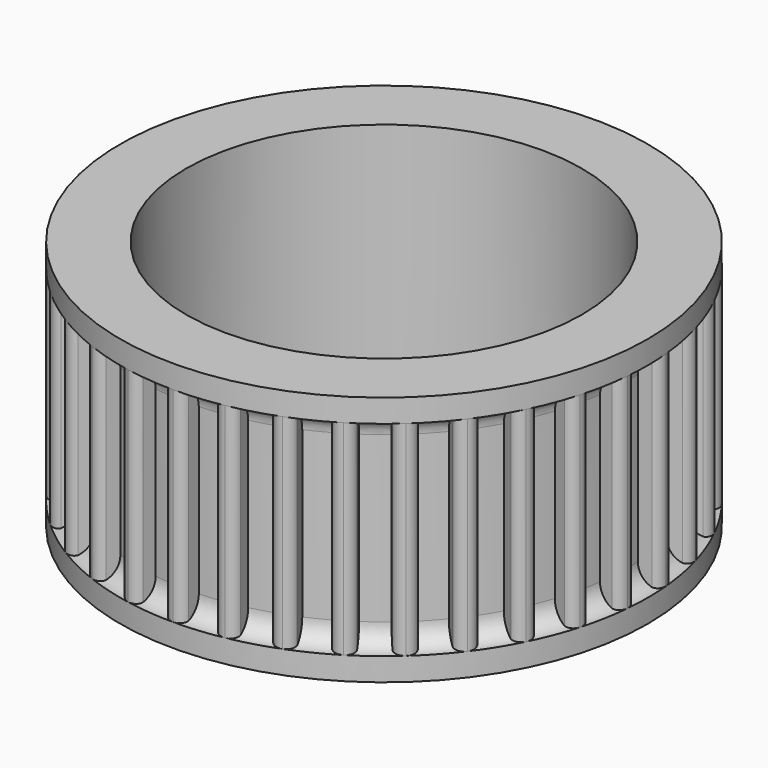
from build123d import *

# Parameters (mm, degrees)
F0_R             = 20
F1_DEPTH         = 19
F2_W             = 1.5
F2_H             = 15.5
F5_R             = 1.49999
F4_W             = 1.5
F4_H             = 19.3690806627
F6_DEPTH         = 19
F6_COPIES_COUNT  = 34
F6_COPIES1_COUNT = 2
F6_COPIES1_ANGLE = 84.7059
F6_COPIES2_COUNT = 2
F6_COPIES2_ANGLE = 95.2941
F6_COPIES3_COUNT = 2
F6_COPIES3_ANGLE = 275.2941
F7_R             = 15
F8_DEPTH         = 19.001


# Not quite as in the source:
# - a fillet or chamfer is up to 0.001 mm smaller than in the source, because OpenCascade refuses the exact size
# - a pattern or mirror of a feature is missing from the dataset's text; its kind, count and spacing are read off the source's solid


with BuildPart() as f1:
    # F0 (on Top) → F1 (new body)
    with BuildSketch(Plane.XY):
        Circle(F0_R)
    extrude(amount=F1_DEPTH)

    # F2 (on Front) → F3 (revolve, cut)
    with BuildSketch(Plane.XZ):
        with Locations((-19.25, 9.5)):
            Rectangle(F2_W, F2_H)
    revolve(axis=Axis((0, 0, 23.3165337704), (0, 0, -1)), mode=Mode.SUBTRACT)

    # F5 (radius 1.5 in the source; OpenCascade refuses exactly that, so slightly less here)
    f5_edges = [f1.edges().sort_by_distance(p)[0] for p in [
        (18.5, 0, 17.25),
        (18.5, 0, 1.75),
    ]]
    fillet(f5_edges, radius=F5_R)

    # F4 (on face) → F6 (join)
    with BuildSketch(Plane.XY.offset(19)):
        with BuildLine():
            Line((-0.75, 19.4735489786), (-0.75, 19.3690806627))
            Line((-0.75, 19.3690806627), (0.75, 19.3690806627))
            Line((0.75, 19.3690806627), (0.75, 19.4735489786))
            ThreePointArc((0.75, 19.4735489786), (0.4581622742, 19.8552502887), (0, 20))
            ThreePointArc((0, 20), (-0.4581622742, 19.8552502887), (-0.75, 19.4735489786))
        make_face()
        with Locations((0, 9.6845403314)):
            Rectangle(F4_W, F4_H)
    f6 = extrude(amount=-F6_DEPTH)

    # F6_copies: F6 ×34 about axis
    f6_copies_axis = Axis((0, 0, 0), (0, 0, 1))
    for i in range(1, F6_COPIES_COUNT):
        add(f6.rotate(f6_copies_axis, i * 360 / F6_COPIES_COUNT))

    # F6_copies1: F6 ×2 about axis
    f6_copies1_axis = Axis((0, 0, 0), (0, 0, 1))
    for i in range(1, F6_COPIES1_COUNT):
        add(f6.rotate(f6_copies1_axis, i * F6_COPIES1_ANGLE / (F6_COPIES1_COUNT - 1)))

    # F6_copies2: F6 ×2 about axis
    f6_copies2_axis = Axis((0, 0, 0), (0, 0, 1))
    for i in range(1, F6_COPIES2_COUNT):
        add(f6.rotate(f6_copies2_axis, i * F6_COPIES2_ANGLE / (F6_COPIES2_COUNT - 1)))

    # F6_copies3: F6 ×2 about axis
    f6_copies3_axis = Axis((0, 0, 0), (0, 0, 1))
    for i in range(1, F6_COPIES3_COUNT):
        add(f6.rotate(f6_copies3_axis, i * F6_COPIES3_ANGLE / (F6_COPIES3_COUNT - 1)))

    # F7 (on face) → F8 (cut, through all)
    with BuildSketch(Plane.XY.offset(19)):
        Circle(F7_R)
    extrude(amount=-F8_DEPTH, mode=Mode.SUBTRACT)


solid = f1.part
